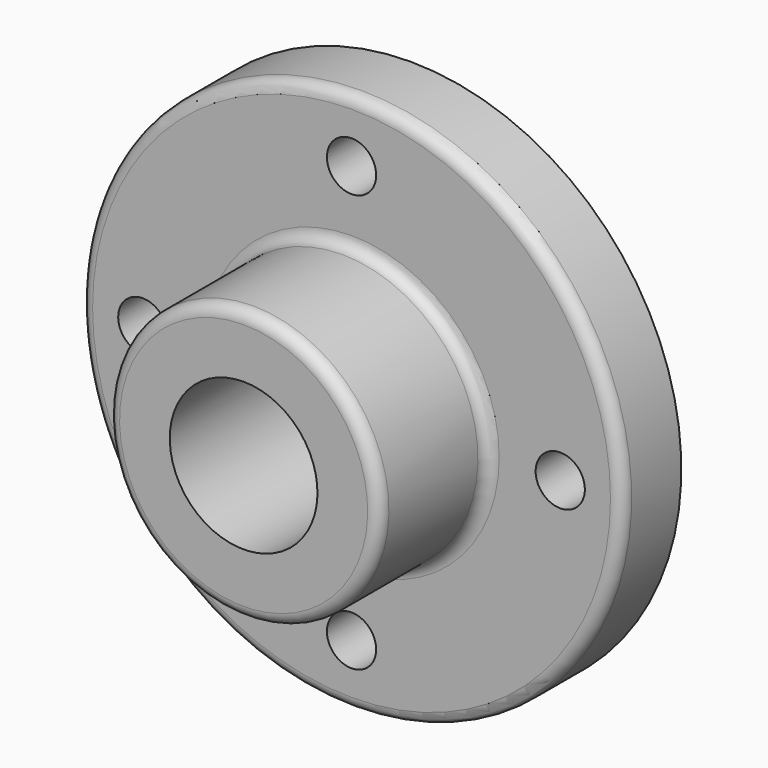
from build123d import *

# Parameters (mm, degrees)
F2_R            = 3.048
F3_R            = 6.35
F4_DEPTH        = 19.051
F4_COPIES_COUNT = 4


# Not quite as in the source:
# - a pattern or mirror of a feature is missing from the dataset's text; its kind, count and spacing are read off the source's solid


with BuildPart() as f1:
    # F0 (on Right) → F1 (revolve)
    with BuildSketch(Plane.YZ):
        Polygon((-53.848, 19.05), (0, 19.05), (0, 69.85), (-19.05, 69.85), (-19.05, 35.052), (-53.848, 35.052), align=None)
    revolve(axis=Axis((0, -31.5901881313, 0), (0, -1, 0)))

    # F2
    f2_edges = [f1.edges().sort_by_distance(p)[0] for p in [
        (0, -53.848, -35.052),
        (0, -19.05, -35.052),
        (0, -19.05, -69.85),
    ]]
    fillet(f2_edges, radius=F2_R)

    # F3 (on face) → F4 (cut, through all)
    with BuildSketch(Plane.XZ.offset(19.05)):
        with Locations((0, 53.848)):
            Circle(F3_R)
    f4 = extrude(amount=-F4_DEPTH, mode=Mode.SUBTRACT)

    # F4_copies: F4 ×4 about axis
    f4_copies_axis = Axis((0, 0, 0), (0, 1, 0))
    for i in range(1, F4_COPIES_COUNT):
        add(f4.rotate(f4_copies_axis, i * 360 / F4_COPIES_COUNT), mode=Mode.SUBTRACT)


solid = f1.part
